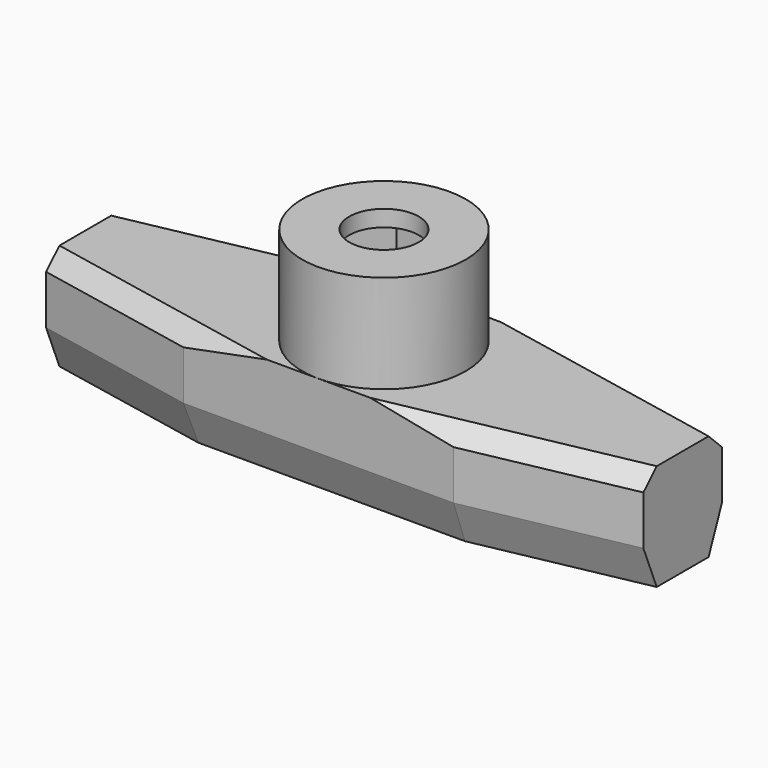
from build123d import *

# Parameters (mm, degrees)
F1_DEPTH    = 13
F3_DEPTH    = 3.2
F4_R        = 4.25
F5_DEPTH    = 13
F6_C1_SIZE2 = 2
F6_C1_SIZE  = 5
F6_C2_SIZE2 = 2
F6_C2_SIZE  = 5
F6_C3_SIZE2 = 5
F6_C3_SIZE  = 2
F6_C4_SIZE2 = 5
F6_C4_SIZE  = 2
F6_C5_SIZE2 = 5
F6_C5_SIZE  = 2
F6_C6_SIZE2 = 5
F6_C6_SIZE  = 2
F7_SIZE     = 2
F9_R        = 10
F9_R_2      = 4.25
F10_DEPTH   = 12
F11_R       = 4.25
F12_DEPTH   = 10


with BuildPart() as f1:
    # F0 (on Top) → F1 (new body)
    with BuildSketch(Plane.XY):
        Polygon((-16.5, -10), (16.5, -10), (36.5, -6), (36.5, 6), (16.5, 10), (-16.5, 10), (-36.5, 6), (-36.5, -6), align=None)
    extrude(amount=F1_DEPTH)

    # F2 (on face) → F3 (join)
    with BuildSketch(Plane.XY.offset(13)):
        Polygon((-3.7527767497, -6.5), (3.7527767497, -6.5), (7.5055534995, 0), (3.7527767497, 6.5), (-3.7527767497, 6.5), (-7.5055534995, 0), align=None)
    extrude(amount=F3_DEPTH)

    # F4 (on face) → F5 (cut)
    with BuildSketch(Plane.XY.offset(16.2)):
        Circle(F4_R)
    extrude(amount=-F5_DEPTH, mode=Mode.SUBTRACT)

    # F6: chamfer of 5 x 2 on 6 edges, made by hand

    # F6_c1
    f6_c1_edges = [f1.edges().sort_by_distance(p)[0] for p in [
        (0, -10, 0),
    ]]
    f6_c1_side = f1.faces().sort_by_distance((0, -10, 0.04))[0]
    chamfer(f6_c1_edges, length=F6_C1_SIZE, length2=F6_C1_SIZE2, reference=f6_c1_side)

    # F6_c2
    f6_c2_edges = [f1.edges().sort_by_distance(p)[0] for p in [
        (-31.5, -7, 0),
    ]]
    f6_c2_side = f1.faces().sort_by_distance((-31.5, -7, 0.04))[0]
    chamfer(f6_c2_edges, length=F6_C2_SIZE, length2=F6_C2_SIZE2, reference=f6_c2_side)

    # F6_c3
    f6_c3_edges = [f1.edges().sort_by_distance(p)[0] for p in [
        (31.5, -7, 0),
    ]]
    f6_c3_side = f1.faces().sort_by_distance((31.4921553546, -6.960776773, 0))[0]
    chamfer(f6_c3_edges, length=F6_C3_SIZE, length2=F6_C3_SIZE2, reference=f6_c3_side)

    # F6_c4
    f6_c4_edges = [f1.edges().sort_by_distance(p)[0] for p in [
        (26.5, 8, 0),
    ]]
    f6_c4_side = f1.faces().sort_by_distance((26.4921553546, 7.960776773, 0))[0]
    chamfer(f6_c4_edges, length=F6_C4_SIZE, length2=F6_C4_SIZE2, reference=f6_c4_side)

    # F6_c5
    f6_c5_edges = [f1.edges().sort_by_distance(p)[0] for p in [
        (-5.0990195136, 10, 0),
    ]]
    f6_c5_side = f1.faces().sort_by_distance((-5.0990195136, 9.96, 0))[0]
    chamfer(f6_c5_edges, length=F6_C5_SIZE, length2=F6_C5_SIZE2, reference=f6_c5_side)

    # F6_c6
    f6_c6_edges = [f1.edges().sort_by_distance(p)[0] for p in [
        (-31.5, 7, 0),
    ]]
    f6_c6_side = f1.faces().sort_by_distance((-31.4921553546, 6.960776773, 0))[0]
    chamfer(f6_c6_edges, length=F6_C6_SIZE, length2=F6_C6_SIZE2, reference=f6_c6_side)

    # F7
    f7_edges = [f1.edges().sort_by_distance(p)[0] for p in [
        (26.5, -8, 13),
        (26.5, 8, 13),
        (-26.5, 8, 13),
        (-26.5, -8, 13),
    ]]
    chamfer(f7_edges, length=F7_SIZE)


with BuildPart() as f10:
    # F9 (on offset) → F10 (new body)
    with BuildSketch(Plane.XY.offset(25)):
        Circle(F9_R)
        Circle(F9_R_2, mode=Mode.SUBTRACT)
    extrude(amount=-F10_DEPTH)

    # F11 (on face) → F12 (cut)
    with BuildSketch(Plane(origin=(0, 0, 13), x_dir=(1, 0, 0), z_dir=(0, 0, -1))):
        Polygon((-3.897114317, -6.75), (3.897114317, -6.75), (7.7942286341, 0), (3.897114317, 6.75), (-3.897114317, 6.75), (-7.7942286341, 0), align=None)
        Circle(F11_R, mode=Mode.SUBTRACT)
    extrude(amount=-F12_DEPTH, mode=Mode.SUBTRACT)


solid = Compound([f1.part, f10.part])
